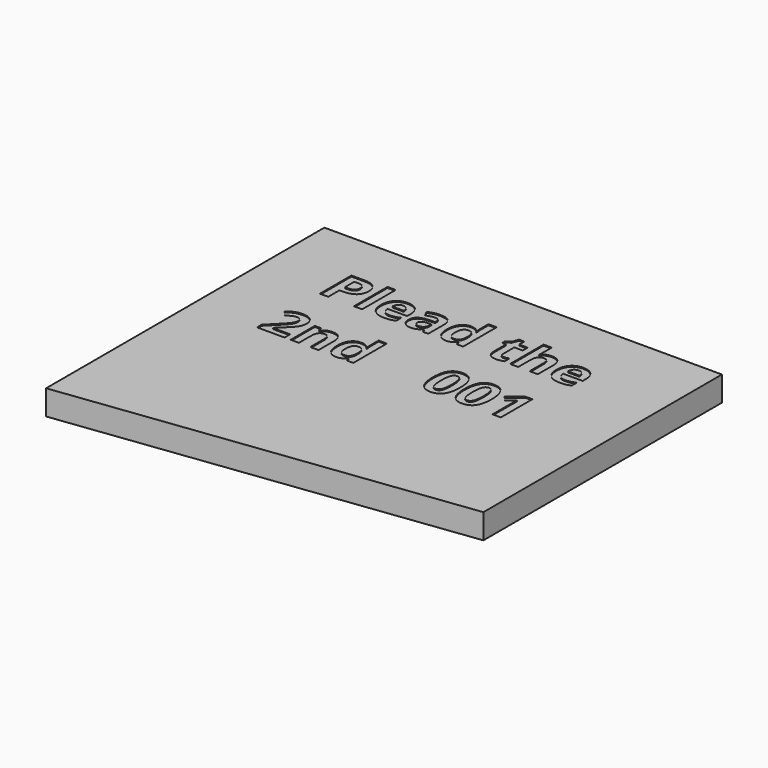
from build123d import *

# Parameters (mm, degrees)
F1_DEPTH     = 3.175
F2_TEXT_SIZE = 7.2190220012
F3_DEPTH     = 0.0762
F4_TEXT_SIZE = 7.0562555809
F5_DEPTH     = 0.127


# Not quite as in the source:
# - Text() gives the source's letters only with a copy of the font that has no kerning and outlines rounded to 1/6400 em; it was checked with that copy


with BuildPart() as f1:
    # F0 (on Top) → F1 (new body)
    with BuildSketch(Plane.XY):
        Polygon((-6.35, -3.175), (-57.15, -3.175), (-57.15, -47.625), (-6.35, -41.275), align=None)
    extrude(amount=F1_DEPTH)

    # F2 (on face) → F3 (cut)
    with BuildSketch(Plane.XY.offset(3.175)):
        with Locations((-22.3182930972, 11.9338437947)):
            Text('Plead the 2nd', F2_TEXT_SIZE, font='Open Sans', font_style=FontStyle.ITALIC, text_align=(TextAlign.LEFT, TextAlign.BOTTOM))
    extrude(amount=-F3_DEPTH, mode=Mode.SUBTRACT)

    # F4 (on face) → F5 (cut)
    with BuildSketch(Plane.XY.offset(3.175)):
        with Locations((-49.2125, -14.6055040183)):
            Text('Plead the', F4_TEXT_SIZE, font='Open Sans', font_style=FontStyle.BOLD, text_align=(TextAlign.LEFT, TextAlign.BOTTOM))
        with Locations((-49.2125, -24.2020116083)):
            Text('2nd    001', F4_TEXT_SIZE, font='Open Sans', font_style=FontStyle.BOLD, text_align=(TextAlign.LEFT, TextAlign.BOTTOM))
    extrude(amount=-F5_DEPTH, mode=Mode.SUBTRACT)


solid = f1.part
